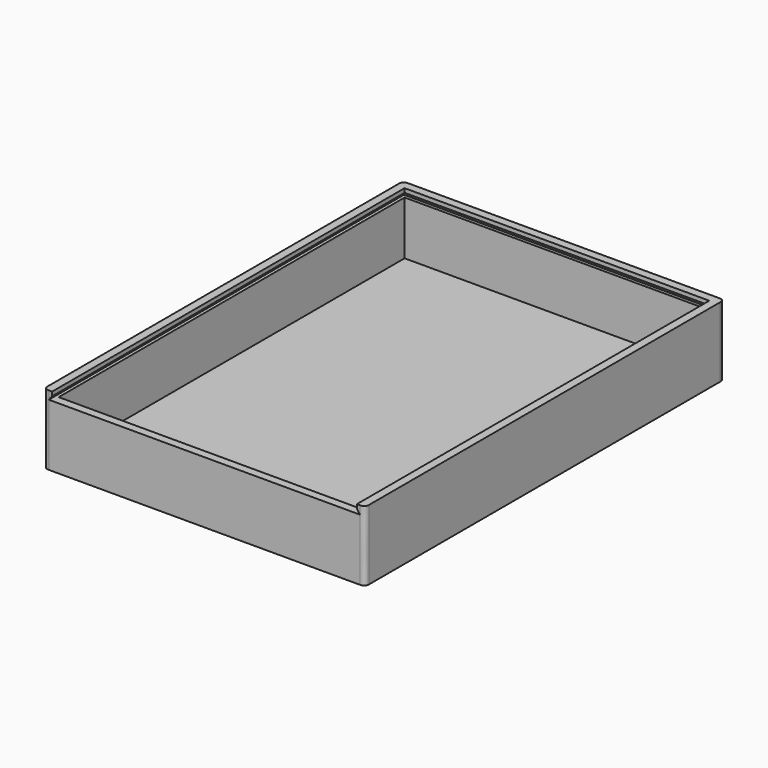
from build123d import *

# Parameters (mm, degrees)
F0_W        = 78
F0_H        = 15
F1_DEPTH    = 109
F2_T        = -2
F4_DEPTH    = 109
F6_DEPTH    = 78
F7_T1_DEPTH = 23


# Not quite as in the source:
# - a fillet or chamfer that OpenCascade refuses, or shapes differently, is made with other operations: its cross-section is extruded or revolved along the edge and cut away or added


with BuildPart() as f1:
    # F0 (on Front) → F1 (new body)
    with BuildSketch(Plane.XZ):
        with Locations((39, -7.5)):
            Rectangle(F0_W, F0_H)
    extrude(amount=-F1_DEPTH)

    # F2
    f2_openings = [f1.faces().sort_by_distance(p)[0] for p in [
        (39, 54.5, 0),
    ]]
    offset(amount=F2_T, openings=f2_openings)

    # F3 (on face) → F4 (join, through all)
    with BuildSketch(Plane.XZ):
        Polygon((0, 2), (0, 0), (1.2, 0), (2, 1), (2, 2), align=None)
        Polygon((76, 1), (76.8, 0), (78, 0), (78, 2), (76, 2), align=None)
    extrude(amount=-F4_DEPTH)

    # F5 (on face) → F6 (join, through all)
    with BuildSketch(Plane.YZ.offset(78)):
        Polygon((109, 0), (109, 2), (107, 2), (107, 1), (107.8, 0), align=None)
    extrude(amount=-F6_DEPTH)

    # F7: fillet of radius 1.2 on 4 edges, made by hand

    # F7_s2 → F7_t1 (cut)
    with BuildSketch(Plane.XY.offset(-18)):
        with BuildLine():
            add(Edge.make_bspline(
                [(78, 1.2), (78, 0), (76.8, 0)],
                knots=[0, 0, 0, 1, 1, 1], degree=2, weights=[1, 1, 1]))
            Line((76.8, 0), (78, 0))
            Line((78, 0), (78, 1.2))
        make_face()
        with BuildLine():
            add(Edge.make_bspline(
                [(76.8, 109), (78, 109), (78, 107.8)],
                knots=[0, 0, 0, 1, 1, 1], degree=2, weights=[1, 1, 1]))
            Line((78, 107.8), (78, 109))
            Line((78, 109), (76.8, 109))
        make_face()
        with BuildLine():
            add(Edge.make_bspline(
                [(0, 107.8), (0, 109), (1.2, 109)],
                knots=[0, 0, 0, 1, 1, 1], degree=2, weights=[1, 1, 1]))
            Line((1.2, 109), (0, 109))
            Line((0, 109), (0, 107.8))
        make_face()
        with BuildLine():
            add(Edge.make_bspline(
                [(0, 1.2), (0, 0), (1.2, 0)],
                knots=[0, 0, 0, 1, 1, 1], degree=2, weights=[1, 1, 1]))
            Line((1.2, 0), (0, 0))
            Line((0, 0), (0, 1.2))
        make_face()
    extrude(amount=F7_T1_DEPTH, mode=Mode.SUBTRACT)


solid = f1.part
